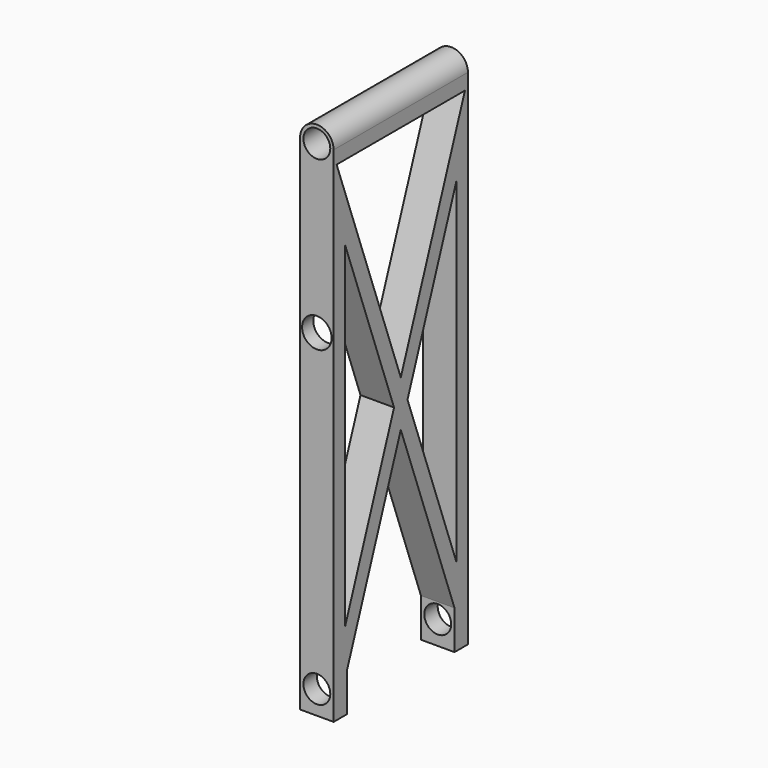
from build123d import *

# Parameters (mm, degrees)
F1_DEPTH = 6.35
F3_DEPTH = 2.54
F4_W     = 10.16
F4_H     = 2.9410431877
F5_DEPTH = 2.54
F6_R     = 1.016
F7_DEPTH = 12.7
F8_R     = 1.1176
F9_DEPTH = 2.54


# Not quite as in the source:
# - a feature names something its author has since deleted; it is built from what else it names


with BuildPart() as f1:
    # F0 (on Front) → F1 (new body, symmetric)
    with BuildSketch(Plane.XZ):
        with BuildLine():
            Line((1.27, -38.1), (1.27, 0))
            ThreePointArc((1.27, 0), (0.8980256121, 0.8980256121), (0, 1.27))
            ThreePointArc((0, 1.27), (-0.8980256121, 0.8980256121), (-1.27, 0))
            Line((-1.27, 0), (-1.27, -38.1))
            Line((-1.27, -38.1), (1.27, -38.1))
        make_face()
    extrude(amount=F1_DEPTH, both=True)

    # F2 (on face) → F3 (cut)
    with BuildSketch(Plane.YZ.offset(1.27)):
        Polygon((0.635, -19.4826158311), (5.2897260698, -32.2506076148), (5.2897260698, -6.7146240474), align=None)
        Polygon((0, -35.1589568123), (5.08, -35.1589568123), (0, -21.2244314957), align=None)
        Polygon((0, -1.0980047432), (0, -17.7408001665), (6.067332674, -1.0980047432), align=None)
        Polygon((-6.067332674, -1.0980047432), (0, -17.7408001665), (0, -1.0980047432), align=None)
        Polygon((0, -35.1589568123), (0, -21.2244314957), (-5.08, -35.1589568123), align=None)
        Polygon((-5.2897260698, -32.2506076148), (-0.635, -19.4826158311), (-5.2897260698, -6.7146240474), align=None)
    extrude(amount=-F3_DEPTH, mode=Mode.SUBTRACT)

    # F4 (on face) → F5 (cut)
    with BuildSketch(Plane.YZ.offset(1.27)):
        with Locations((0, -36.6294784061)):
            Rectangle(F4_W, F4_H)
    extrude(amount=-F5_DEPTH, mode=Mode.SUBTRACT)

    # F6 (on face) → F7 (cut)
    with BuildSketch(Plane.XZ.offset(6.35)):
        with Locations((0, -36.322)):
            Circle(F6_R)
        Circle(F6_R)
    extrude(amount=-F7_DEPTH, mode=Mode.SUBTRACT)

    # F8 (on face) → F9 (cut)
    with BuildSketch(Plane.XZ.offset(6.35)):
        with Locations((0, -12.589443475)):
            Circle(F8_R)
    extrude(amount=-F9_DEPTH, mode=Mode.SUBTRACT)


solid = f1.part
